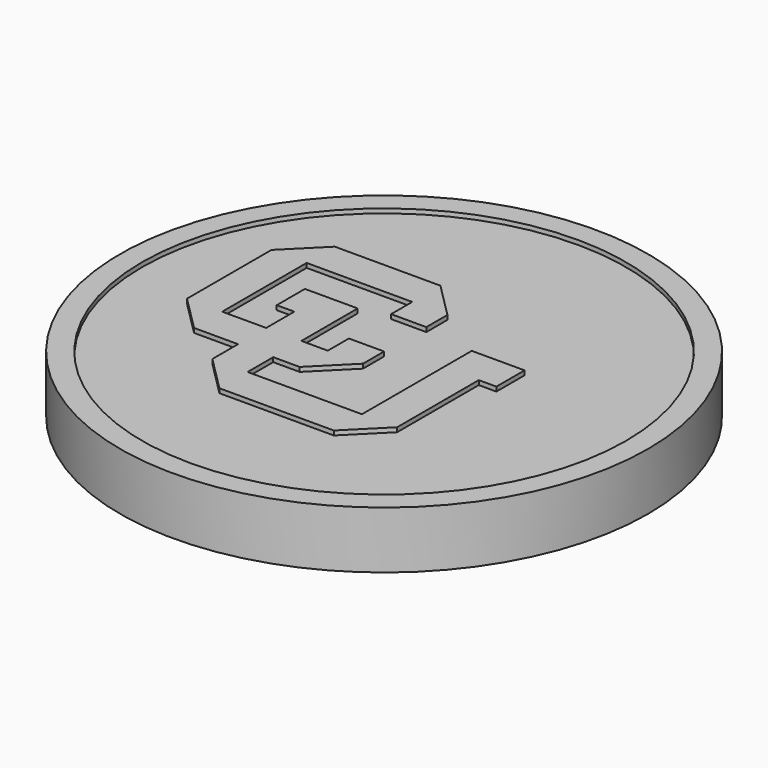
from build123d import *

# Parameters (mm, degrees)
F0_R         = 38.1
F1_DEPTH     = 3.81
F3_R         = 38.1
F3_R_2       = 34.925
F4_DEPTH     = 4.445
F6_TEXT_SIZE = 21.1666666667
F5_R         = 38.1
F5_R_2       = 34.925
F7_DEPTH     = 3.81


# Not quite as in the source:
# - Text() gives the source's letters only with a copy of the font that has no kerning and outlines rounded to 1/6400 em; it was checked with that copy


with BuildPart() as f1:
    # F0 (on Top) → F1 (new body)
    with BuildSketch(Plane.XY):
        Circle(F0_R)
    extrude(amount=F1_DEPTH)

    # F3 (on Top) + F2 (on Top) → F4 (join)
    with BuildSketch(Plane.XY):
        Circle(F3_R)
        Circle(F3_R_2, mode=Mode.SUBTRACT)
    with BuildSketch(Plane.XY):
        Polygon((0, -3.81), (0, 0), (-5.08, 0), (-5.08, -3.81), (-8.89, -3.81), (-8.89, 6.35), (-16.51, 6.35), (-16.51, 1.27), (-13.97, 1.27), (-13.97, -3.81), (-20.32, -3.81), (-20.32, 11.43), (-5.08, 11.43), (-5.08, 7.62), (0, 7.62), (0, 11.43), (-5.08, 16.51), (-20.32, 16.51), (-25.4, 11.43), (-25.4, -3.81), (-20.32, -8.89), (-13.97, -8.89), (-13.97, -13.5191705856), (-8.89, -18.5991705856), (7.62, -18.5991705856), (12.7, -13.5191705856), (12.7, 1.2128294144), (15.24, 1.2128294144), (15.24, 6.2928294144), (7.62, 6.2928294144), (7.62, -13.5191705856), (-8.89, -13.5191705856), (-8.89, -8.89), (-5.08, -8.89), align=None)
    extrude(amount=F4_DEPTH)

    # F6 (on face) + F5 (on face) → F7 (join)
    with BuildSketch(Plane(origin=(0, 0, 0), x_dir=(1, 0, 0), z_dir=(0, 0, -1))):
        with Locations((-23.839657881, 5.2535466709)):
            Text('Alan', F6_TEXT_SIZE, font='Open Sans', text_align=(TextAlign.LEFT, TextAlign.BOTTOM))
        with Locations((-23.839657881, -23.5331199958)):
            Text('PV', F6_TEXT_SIZE, font='Open Sans', text_align=(TextAlign.LEFT, TextAlign.BOTTOM))
    with BuildSketch(Plane(origin=(0, 0, 0), x_dir=(1, 0, 0), z_dir=(0, 0, -1))):
        Circle(F5_R)
        Circle(F5_R_2, mode=Mode.SUBTRACT)
    extrude(amount=F7_DEPTH)


solid = f1.part
